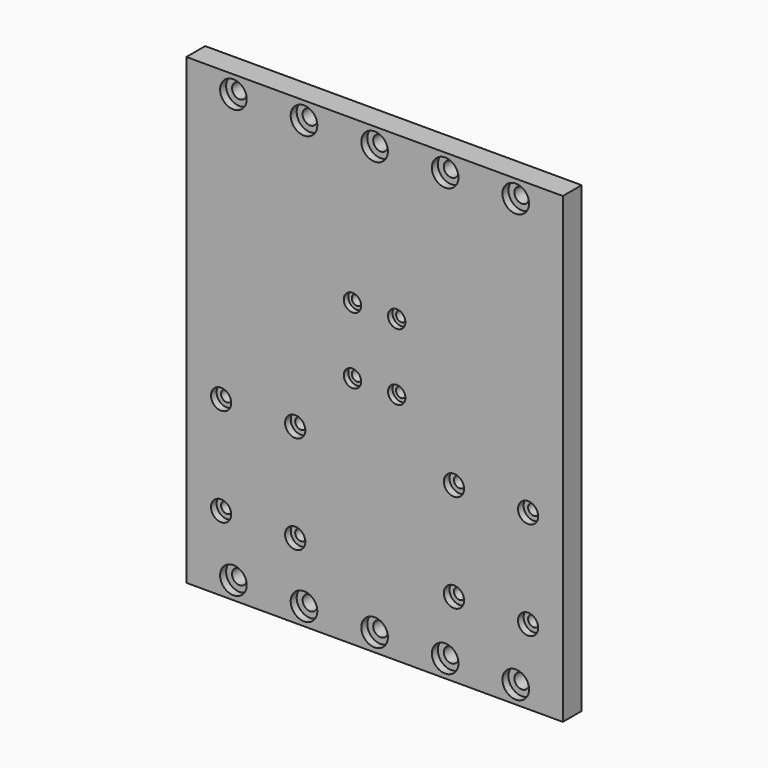
from build123d import *

# Parameters (mm, degrees)
F0_W      = 203.2
F0_H      = 249.9106
F0_R      = 2.794
F1_DEPTH  = 12.7
F2_R      = 4.0005
F3_DEPTH  = 12.701
F4_R      = 3.048
F5_DEPTH  = 12.701
F6_DEPTH  = 329
F7_R      = 7.1882
F8_DEPTH  = 4.064
F9_R      = 4.699
F10_DEPTH = 3.048
F11_R     = 5.461
F12_DEPTH = 3.81


# Not quite as in the source:
# - an extrude ends at something that could not be found from the text; its depth is read off the source's solid


with BuildPart() as f1:
    # F0 (on Front) → F1 (new body)
    with BuildSketch(Plane.XZ):
        Rectangle(F0_W, F0_H)
        with Locations((-11.938, 1.3843)):
            Circle(F0_R, mode=Mode.SUBTRACT)
        with Locations((-11.938, 37.3761)):
            Circle(F0_R, mode=Mode.SUBTRACT)
        with Locations((11.938, 1.3843)):
            Circle(F0_R, mode=Mode.SUBTRACT)
        with Locations((11.938, 37.3761)):
            Circle(F0_R, mode=Mode.SUBTRACT)
    extrude(amount=F1_DEPTH)

    # F2 (on face) → F3 (cut, through all)
    with BuildSketch(Plane.XZ.offset(12.7)):
        with Locations((-76.2, 115.4303)):
            Circle(F2_R)
        with Locations((-38.1, 115.4303)):
            Circle(F2_R)
        with Locations((0, 115.4303)):
            Circle(F2_R)
        with Locations((38.1, 115.4303)):
            Circle(F2_R)
        with Locations((76.2, 115.4303)):
            Circle(F2_R)
        with Locations((-76.2, -115.4303)):
            Circle(F2_R)
        with Locations((-38.1, -115.4303)):
            Circle(F2_R)
        with Locations((0, -115.4303)):
            Circle(F2_R)
        with Locations((38.1, -115.4303)):
            Circle(F2_R)
        with Locations((76.2, -115.4303)):
            Circle(F2_R)
    extrude(amount=-F3_DEPTH, mode=Mode.SUBTRACT)

    # F4 (on face) → F5 (cut, through all)
    with BuildSketch(Plane(origin=(0, 0, 0), x_dir=(-1, 0, 0), z_dir=(0, 1, 0))):
        with Locations((82.8548, -31.57982)):
            Circle(F4_R)
        with Locations((42.8498, -31.57982)):
            Circle(F4_R)
        with Locations((82.8548, -84.58962)):
            Circle(F4_R)
        with Locations((42.8498, -84.58962)):
            Circle(F4_R)
        with Locations((-42.8498, -31.57982)):
            Circle(F4_R)
        with Locations((-82.8548, -31.57982)):
            Circle(F4_R)
        with Locations((-82.8548, -84.58962)):
            Circle(F4_R)
        with Locations((-42.8498, -84.58962)):
            Circle(F4_R)
    extrude(amount=-F5_DEPTH, mode=Mode.SUBTRACT)

    # F0 (on Front) → F6 (cut, through all)
    with BuildSketch(Plane.XZ):
        Rectangle(F0_W, F0_H)
        with Locations((-11.938, 1.3843)):
            Circle(F0_R, mode=Mode.SUBTRACT)
        with Locations((-11.938, 37.3761)):
            Circle(F0_R, mode=Mode.SUBTRACT)
        with Locations((11.938, 1.3843)):
            Circle(F0_R, mode=Mode.SUBTRACT)
        with Locations((11.938, 37.3761)):
            Circle(F0_R, mode=Mode.SUBTRACT)
    extrude(amount=-F6_DEPTH, mode=Mode.SUBTRACT)

    # F7 (on face) → F8 (cut)
    with BuildSketch(Plane.XZ.offset(12.7)):
        with Locations((-76.2, -115.4303)):
            Circle(F7_R)
        with Locations((-38.1, -115.4303)):
            Circle(F7_R)
        with Locations((0, -115.4303)):
            Circle(F7_R)
        with Locations((38.1, -115.4303)):
            Circle(F7_R)
        with Locations((76.2, -115.4303)):
            Circle(F7_R)
        with Locations((-76.2, 115.4303)):
            Circle(F7_R)
        with Locations((-38.1, 115.4303)):
            Circle(F7_R)
        with Locations((0, 115.4303)):
            Circle(F7_R)
        with Locations((38.1, 115.4303)):
            Circle(F7_R)
        with Locations((76.2, 115.4303)):
            Circle(F7_R)
    extrude(amount=-F8_DEPTH, mode=Mode.SUBTRACT)

    # F9 (on face) → F10 (cut)
    with BuildSketch(Plane.XZ.offset(12.7)):
        with Locations((-11.938, 37.3761)):
            Circle(F9_R)
        with Locations((11.938, 37.3761)):
            Circle(F9_R)
        with Locations((11.938, 1.3843)):
            Circle(F9_R)
        with Locations((-11.938, 1.3843)):
            Circle(F9_R)
    extrude(amount=-F10_DEPTH, mode=Mode.SUBTRACT)

    # F11 (on face) → F12 (cut)
    with BuildSketch(Plane.XZ.offset(12.7)):
        with Locations((-82.8548, -31.57982)):
            Circle(F11_R)
        with Locations((-42.8498, -31.57982)):
            Circle(F11_R)
        with Locations((42.8498, -31.57982)):
            Circle(F11_R)
        with Locations((82.8548, -31.57982)):
            Circle(F11_R)
        with Locations((82.8548, -84.58962)):
            Circle(F11_R)
        with Locations((42.8498, -84.58962)):
            Circle(F11_R)
        with Locations((-42.8498, -84.58962)):
            Circle(F11_R)
        with Locations((-82.8548, -84.58962)):
            Circle(F11_R)
    extrude(amount=-F12_DEPTH, mode=Mode.SUBTRACT)


solid = f1.part
